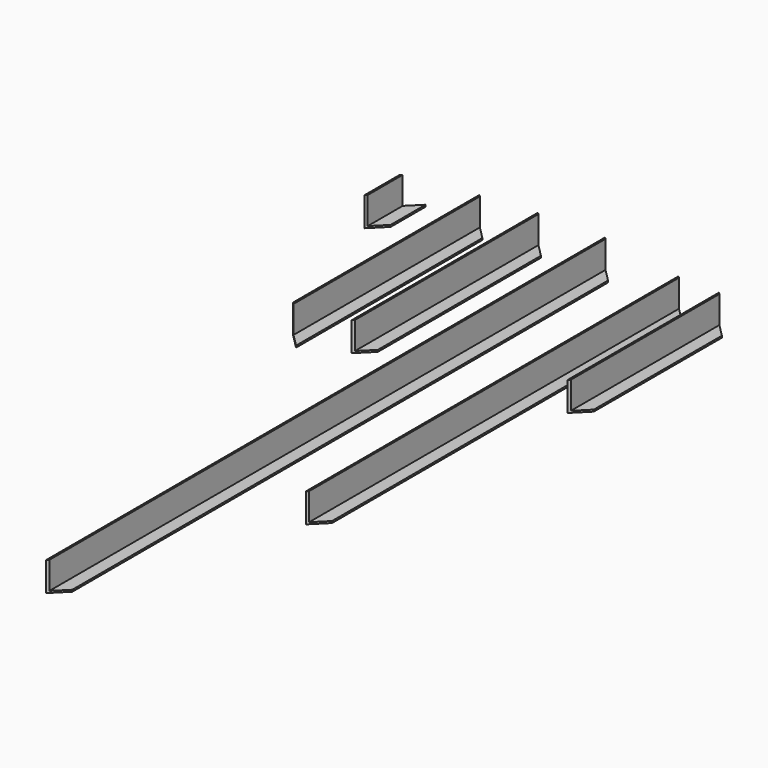
from build123d import *

# Parameters (mm, degrees)
F1_DEPTH  = 1219.2
F3_DEPTH  = 406.4
F4_SIZE   = 25.39999
F4_2_SIZE = 25.39999
F6_DEPTH  = 812.8
F8_DEPTH  = 330.2
F9_SIZE   = 25.39999
F9_2_SIZE = 25.39999
F11_DEPTH = 431.8
F13_DEPTH = 101.6
F14_SIZE  = 25.39999
F15_SIZE  = 25.39999
F16_SIZE  = 25.39999
F17_SIZE  = 25.39999


# Not quite as in the source:
# - a fillet or chamfer is up to 0.001 mm smaller than in the source, because OpenCascade refuses the exact size


with BuildPart() as f1:
    # F0 (on Front) → F1 (new body)
    with BuildSketch(Plane.XZ):
        Polygon((0, 50.8), (0, 0), (25.4, 0), (25.4, 3.175), (3.175, 3.175), (3.175, 50.8), align=None)
    extrude(amount=F1_DEPTH)

    # F4#2 (size 25.4 in the source; OpenCascade refuses exactly that, so slightly less here)
    f4_2_edges = [f1.edges().sort_by_distance(p)[0] for p in [
        (25.4, -1219.2, 1.5875),
        (25.4, 0, 1.5875),
    ]]
    chamfer(f4_2_edges, length=F4_2_SIZE)


with BuildPart() as f3:
    # F2 (on Front) → F3 (new body)
    with BuildSketch(Plane.XZ):
        Polygon((-117.0394197106, 50.8), (-117.0394197106, 0), (-91.6394197106, 0), (-91.6394197106, 3.175), (-113.8644197106, 3.175), (-113.8644197106, 50.8), align=None)
    extrude(amount=F3_DEPTH)

    # F4 (size 25.4 in the source; OpenCascade refuses exactly that, so slightly less here)
    f4_edges = [f3.edges().sort_by_distance(p)[0] for p in [
        (-91.63942, -406.4, 1.5875),
        (-91.63942, 0, 1.5875),
    ]]
    chamfer(f4_edges, length=F4_SIZE)


with BuildPart() as f6:
    # F5 (on Front) → F6 (new body)
    with BuildSketch(Plane.XZ):
        Polygon((128.1303969458, 32.8083333333), (128.1303969458, -17.9916666667), (153.5303969458, -17.9916666667), (153.5303969458, -14.8166666667), (131.3053969458, -14.8166666667), (131.3053969458, 32.8083333333), align=None)
    extrude(amount=F6_DEPTH)

    # F9 (size 25.4 in the source; OpenCascade refuses exactly that, so slightly less here)
    f9_edges = [f6.edges().sort_by_distance(p)[0] for p in [
        (153.530397, 0, -16.404167),
        (153.530397, -812.8, -16.404167),
    ]]
    chamfer(f9_edges, length=F9_SIZE)


with BuildPart() as f8:
    # F7 (on Front) → F8 (new body)
    with BuildSketch(Plane.XZ):
        Polygon((198.6773014069, 30.6892699182), (198.6773014069, -20.1107300818), (224.0773014069, -20.1107300818), (224.0773014069, -16.9357300818), (201.8523014069, -16.9357300818), (201.8523014069, 30.6892699182), align=None)
    extrude(amount=F8_DEPTH)

    # F9#2 (size 25.4 in the source; OpenCascade refuses exactly that, so slightly less here)
    f9_2_edges = [f8.edges().sort_by_distance(p)[0] for p in [
        (224.077301, 0, -18.52323),
        (224.077301, -330.2, -18.52323),
    ]]
    chamfer(f9_2_edges, length=F9_2_SIZE)


with BuildPart() as f11:
    # F10 (on Front) → F11 (new body)
    with BuildSketch(Plane.XZ):
        Polygon((-219.2099541426, 44.7657361247), (-219.2099541426, -6.0342638753), (-193.8099541426, -6.0342638753), (-193.8099541426, -2.8592638753), (-216.0349541426, -2.8592638753), (-216.0349541426, 44.7657361247), align=None)
    extrude(amount=F11_DEPTH)

    # F14 (size 25.4 in the source; OpenCascade refuses exactly that, so slightly less here)
    f14_edges = [f11.edges().sort_by_distance(p)[0] for p in [
        (-219.209954, -431.8, 19.365736),
    ]]
    chamfer(f14_edges, length=F14_SIZE)

    # F15 (size 25.4 in the source; OpenCascade refuses exactly that, so slightly less here)
    f15_edges = [f11.edges().sort_by_distance(p)[0] for p in [
        (-193.809954, 0, -4.446764),
    ]]
    chamfer(f15_edges, length=F15_SIZE)


with BuildPart() as f13:
    # F12 (on Front) → F13 (new body)
    with BuildSketch(Plane.XZ):
        Polygon((-338.6298716068, 46.7442508407), (-338.6298716068, -4.0557491593), (-313.2298716068, -4.0557491593), (-313.2298716068, -0.8807491593), (-335.4548716068, -0.8807491593), (-335.4548716068, 46.7442508407), align=None)
    extrude(amount=F13_DEPTH)

    # F16 (size 25.4 in the source; OpenCascade refuses exactly that, so slightly less here)
    f16_edges = [f13.edges().sort_by_distance(p)[0] for p in [
        (-313.229872, -101.6, -2.468249),
    ]]
    chamfer(f16_edges, length=F16_SIZE)

    # F17 (size 25.4 in the source; OpenCascade refuses exactly that, so slightly less here)
    f17_edges = [f13.edges().sort_by_distance(p)[0] for p in [
        (-338.629872, 0, 21.344251),
    ]]
    chamfer(f17_edges, length=F17_SIZE)


solid = Compound([f1.part, f3.part, f6.part, f8.part, f11.part, f13.part])
